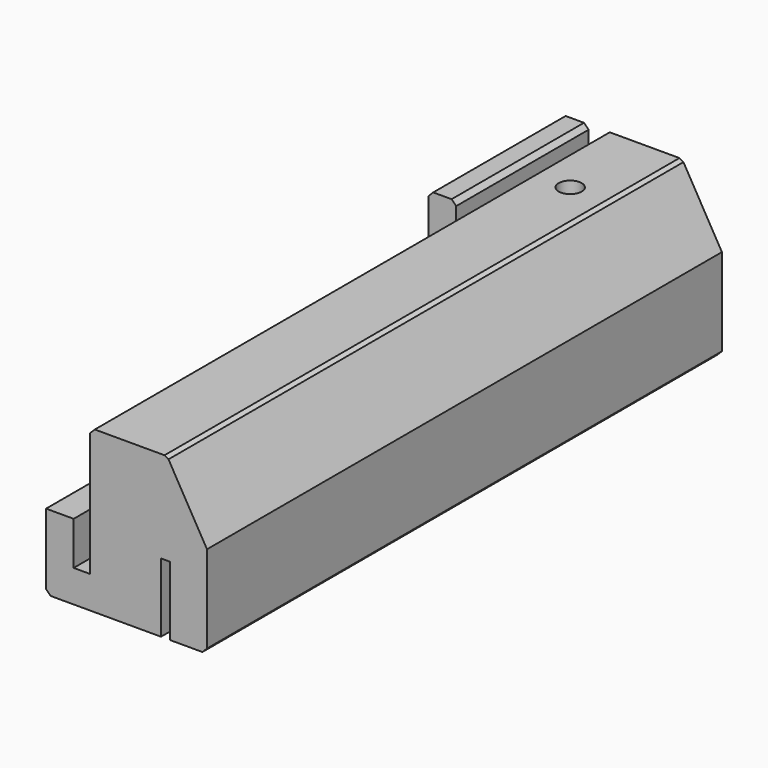
from build123d import *

# Parameters (mm, degrees)
F1_DEPTH        = 177.8
F3_DEPTH        = 9.906
F4_W            = 4.572
F4_H            = 177.8
F5_DEPTH        = 10.16
F7_DEPTH        = 35.56
F9_D            = 8.89
F9_DEPTH        = 5.08
F9_TIP          = 2.6708254516
F10_D           = 6.35
F10_CBORE_D     = 16.51
F10_CBORE_DEPTH = 35.56
F11_T1_DEPTH    = 184.3320747894
F11_T3_DEPTH    = 52.2520747894
F11_T5_DEPTH    = 181.6882193011


# Not quite as in the source:
# - a fillet or chamfer that OpenCascade refuses, or shapes differently, is made with other operations: its cross-section is extruded or revolved along the edge and cut away or added


with BuildPart() as f1:
    # F0 (on Front) → F1 (new body)
    with BuildSketch(Plane.XZ):
        Polygon((0, 44.45), (0, 0), (31.75, 0), (31.75, 19.05), (34.29, 19.05), (34.29, 0), (44.45, 0), (44.45, 25.4), (33.4514773719, 44.45), align=None)
    extrude(amount=F1_DEPTH)

    # F2 (on face) → F3 (cut)
    with BuildSketch(Plane(origin=(0, 0, 0), x_dir=(0, -1, 0), z_dir=(-1, 0, 0))):
        with BuildLine():
            Line((177.8, 20.828), (177.8, 44.45))
            Line((177.8, 44.45), (45.72, 44.45))
            Line((45.72, 44.45), (45.72, 27.178))
            ThreePointArc((45.72, 27.178), (47.5798719395, 22.6878719395), (52.07, 20.828))
            Line((52.07, 20.828), (177.8, 20.828))
        make_face()
    extrude(amount=-F3_DEPTH, mode=Mode.SUBTRACT)

    # F4 (on face) → F5 (cut)
    with BuildSketch(Plane.XY.offset(44.45)):
        with Locations((9.906, -88.9)):
            Rectangle(F4_W, F4_H)
    extrude(amount=-F5_DEPTH, mode=Mode.SUBTRACT)

    # F6 (on face) → F7 (cut)
    with BuildSketch(Plane.XY.offset(44.45)):
        with BuildLine():
            Line((7.62, -177.8), (12.192, -177.8))
            Line((12.192, -177.8), (12.192, -45.72))
            ThreePointArc((12.192, -45.72), (9.906, -43.434), (7.62, -45.72))
            Line((7.62, -45.72), (7.62, -177.8))
        make_face()
    extrude(amount=-F7_DEPTH, mode=Mode.SUBTRACT)

    # F9
    with Locations(Plane(origin=(0, 0, 0), x_dir=(1, 0, 0), z_dir=(0, 0, -1))):
        with Locations((26.67, 38.1)):
            Hole(F9_D / 2, depth=F9_DEPTH)
            with Locations((0, 0, -(F9_DEPTH + F9_TIP / 2))):  # 118° drill point
                Cone(0, F9_D / 2, F9_TIP, mode=Mode.SUBTRACT)

    # F10 (through all)
    with Locations(Plane(origin=(0, 0, 0), x_dir=(1, 0, 0), z_dir=(0, 0, -1))):
        with Locations((22.86, 25.4)):
            CounterBoreHole(F10_D / 2, F10_CBORE_D / 2, F10_CBORE_DEPTH)

    # F11: chamfer of 1.27 on 6 edges, made by hand

    # F11_s2 → F11_t1 (cut)
    with BuildSketch(Plane.XZ.offset(-3.2660373947)):
        Polygon((12.192, 43.18), (13.462, 44.45), (12.192, 44.45), align=None)
        Polygon((0, 1.27), (1.27, 0), (0, 0), align=None)
        Polygon((44.45, 1.27), (43.18, 0), (44.45, 0), align=None)
    extrude(amount=F11_T1_DEPTH, mode=Mode.SUBTRACT)

    # F11_s4 → F11_t3 (cut)
    with BuildSketch(Plane.XZ.offset(-3.2660373947)):
        Polygon((6.35, 44.45), (7.62, 43.18), (7.62, 44.45), align=None)
        Polygon((0, 43.18), (1.27, 44.45), (0, 44.45), align=None)
    extrude(amount=F11_T3_DEPTH, mode=Mode.SUBTRACT)

    # F11_s6 → F11_t5 (cut)
    with BuildSketch(Plane.XZ.offset(-1.9441096505)):
        Polygon((32.7182425301, 44.45), (33.8180947929, 43.815), (33.4514773719, 44.45), align=None)
    extrude(amount=F11_T5_DEPTH, mode=Mode.SUBTRACT)


solid = f1.part
